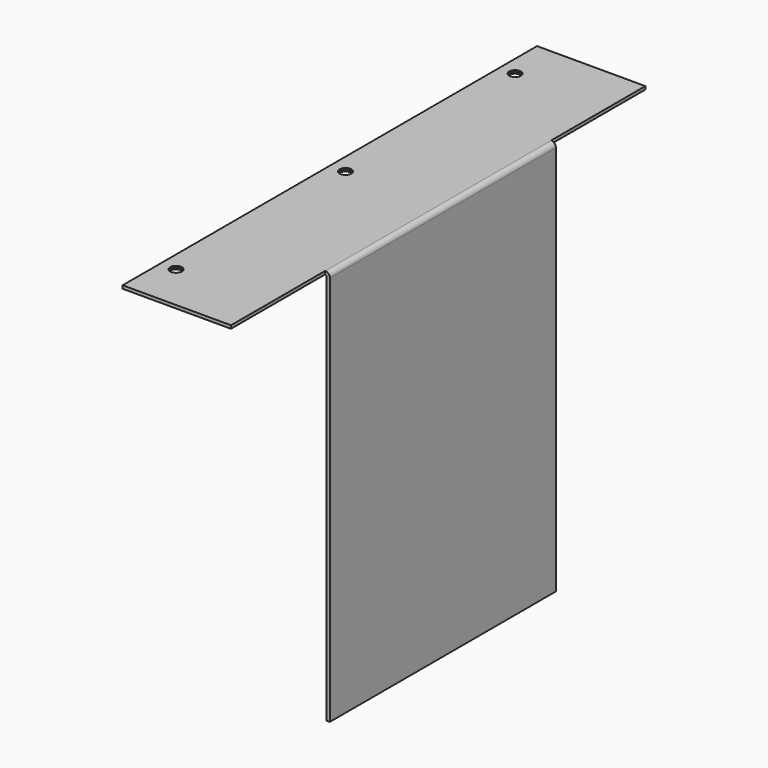
from build123d import *

# Parameters (mm, degrees)
F1_DEPTH = 90
F2_W     = 69
F2_H     = 2
F3_DEPTH = 75
F4_R     = 3.25
F5_DEPTH = 25
F6_SIZE  = 0.5


# Not quite as in the source:
# - a pattern or mirror of a feature is missing from the dataset's text; its kind, count and spacing are read off the source's solid


with BuildPart() as f1:
    # F0 (on Front) → F1 (new body, symmetric)
    with BuildSketch(Plane.XZ):
        with BuildLine():
            ThreePointArc((-1, 0), (-0.2928932188, -0.2928932188), (0, -1))
            Line((0, -1), (0, -250))
            Line((0, -250), (2, -250))
            Line((2, -250), (2, -1))
            ThreePointArc((2, -1), (1.1213203436, 1.1213203436), (-1, 2))
            Line((-1, 2), (-70, 2))
            Line((-70, 2), (-70, 0))
            Line((-70, 0), (-1, 0))
        make_face()
    extrude(amount=F1_DEPTH, both=True)

    # F2 (on face) → F3 (join)
    with BuildSketch(Plane.XZ.offset(90)):
        with Locations((-35.5, 1)):
            Rectangle(F2_W, F2_H)
    f3 = extrude(amount=F3_DEPTH)

    # F3_copies: F3 across plane
    add(f3.mirror(Plane.ZX))

    # F4 (on face) → F5 (cut)
    with BuildSketch(Plane.XY.offset(2)):
        with Locations((-60, 135)):
            Circle(F4_R)
        with Locations((-60, 0)):
            Circle(F4_R)
        with Locations((-60, -135)):
            Circle(F4_R)
    extrude(amount=-F5_DEPTH, mode=Mode.SUBTRACT)

    # F6
    f6_edges = [f1.edges().sort_by_distance(p)[0] for p in [
        (-63.25, 135, 2),
        (-56.75, 135, 1),
        (-63.25, 135, 0),
        (-63.25, 0, 2),
        (-56.75, 0, 1),
        (-63.25, 0, 0),
        (-63.25, -135, 2),
        (-56.75, -135, 1),
        (-63.25, -135, 0),
    ]]
    chamfer(f6_edges, length=F6_SIZE)


solid = f1.part
